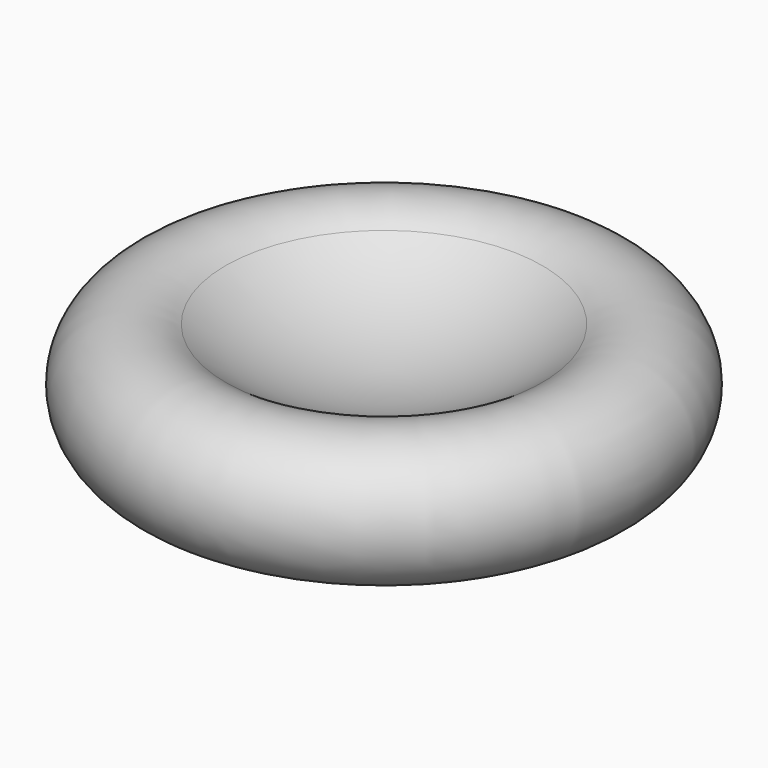
from build123d import *


# Not quite as in the source:
# - the program builds the solid bodies; features that only make, move or delete a surface that nothing else refers to are left out


with BuildPart() as f1:
    # F0 (on Front) → F1 (revolve)
    with BuildSketch(Plane.XZ):
        with BuildLine():
            ThreePointArc((0, 127), (-160.6437051366, 153.0688845903), (-304.8, 228.6))
            ThreePointArc((-304.8, 228.6), (-501.4827788524, 167.1609262841), (-381, 0))
            Line((-381, 0), (0, 0))
            Line((0, 0), (0, 127))
        make_face()
    revolve(axis=Axis((0, 0, 63.5), (0, 0, 1)))


solid = f1.part
